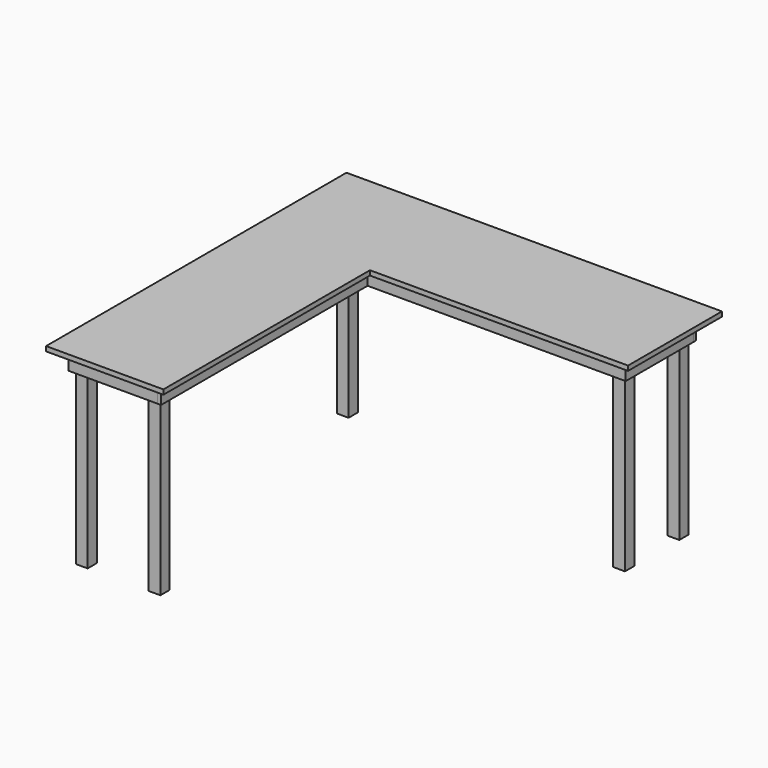
from build123d import *

# Parameters (mm, degrees)
F0_W      = 1100
F0_H      = 500
F1_DEPTH  = 20
F2_W      = 15
F2_H      = 1100
F3_DEPTH  = 75
F4_W      = 15
F4_H      = 75
F5_DEPTH  = 380
F6_W      = 15
F6_H      = 75
F7_DEPTH  = 1460
F8_W      = 15
F8_H      = 75
F9_DEPTH  = 1480
F10_W     = 15
F10_H     = 75
F11_DEPTH = 360
F12_W     = 15
F12_H     = 75
F13_DEPTH = 1465
F14_W     = 50
F14_H     = 50
F15_DEPTH = 800


with BuildPart() as f1:
    # F0 (on Top) → F1 (new body)
    with BuildSketch(Plane.XY):
        Polygon((-277.9552580211, 734.883889217), (-777.9552580211, 734.883889217), (-777.9552580211, -865.116110783), (-277.9552580211, -865.116110783), (-277.9552580211, 234.883889217), align=None)
        with Locations((272.0447419789, 484.883889217)):
            Rectangle(F0_W, F0_H)
    extrude(amount=F1_DEPTH)

    # F4 (on face) → F5 (join)
    with BuildSketch(Plane(origin=(-342.9552580211, 0, 0), x_dir=(0, -1, 0), z_dir=(-1, 0, 0))):
        with Locations((807.616110783, -37.5)):
            Rectangle(F4_W, F4_H)
    extrude(amount=F5_DEPTH)

    # F6 (on face) → F7 (join)
    with BuildSketch(Plane(origin=(0, -800.116110783, 0), x_dir=(-1, 0, 0), z_dir=(0, 1, 0))):
        with Locations((715.4552580211, -37.5)):
            Rectangle(F6_W, F6_H)
    extrude(amount=F7_DEPTH)

    # F10 (on face) → F11 (join)
    with BuildSketch(Plane.XZ.offset(-644.883889217)):
        with Locations((764.5447419789, -37.5)):
            Rectangle(F10_W, F10_H)
    extrude(amount=F11_DEPTH)

    # F12 (on face) → F13 (join, through all)
    with BuildSketch(Plane(origin=(757.0447419789, 0, 0), x_dir=(0, -1, 0), z_dir=(-1, 0, 0))):
        with Locations((-292.383889217, -37.5)):
            Rectangle(F12_W, F12_H)
    extrude(amount=F13_DEPTH)


with BuildPart() as f3:
    # F2 (on Top) → F3 (new body)
    with BuildSketch(Plane.XY):
        with Locations((-335.4552580211, -265.116110783)):
            Rectangle(F2_W, F2_H)
    extrude(amount=-F3_DEPTH)


with BuildPart() as f9:
    # F8 (on face) → F9 (new body)
    with BuildSketch(Plane.YZ.offset(-707.9552580211)):
        with Locations((652.383889217, -37.5)):
            Rectangle(F8_W, F8_H)
    extrude(amount=F9_DEPTH)


with BuildPart() as f15:
    # F14 (on face) → F15 (new body)
    with BuildSketch(Plane(origin=(0, 0, 0), x_dir=(1, 0, 0), z_dir=(0, 0, -1))):
        with Locations((-367.9552580211, 775.116110783)):
            Rectangle(F14_W, F14_H)
    extrude(amount=F15_DEPTH)


with BuildPart() as f16_1:
    # F16: copy of F15
    add(f15.part.moved(Location((-310, 0, 0))))


with BuildPart() as f17_1:
    # F17: copy of F16_1
    add(f16_1.part.moved(Location((0, 1390, 0))))


with BuildPart() as f18_1:
    # F18: copy of F17_1
    add(f17_1.part.moved(Location((1409.5, 0, 0))))


with BuildPart() as f19_1:
    # F19: copy of F18_1
    add(f18_1.part.moved(Location((0, -289.6, 0))))


solid = Compound([f1.part, f3.part, f9.part, f15.part, f16_1.part, f17_1.part, f18_1.part, f19_1.part])
